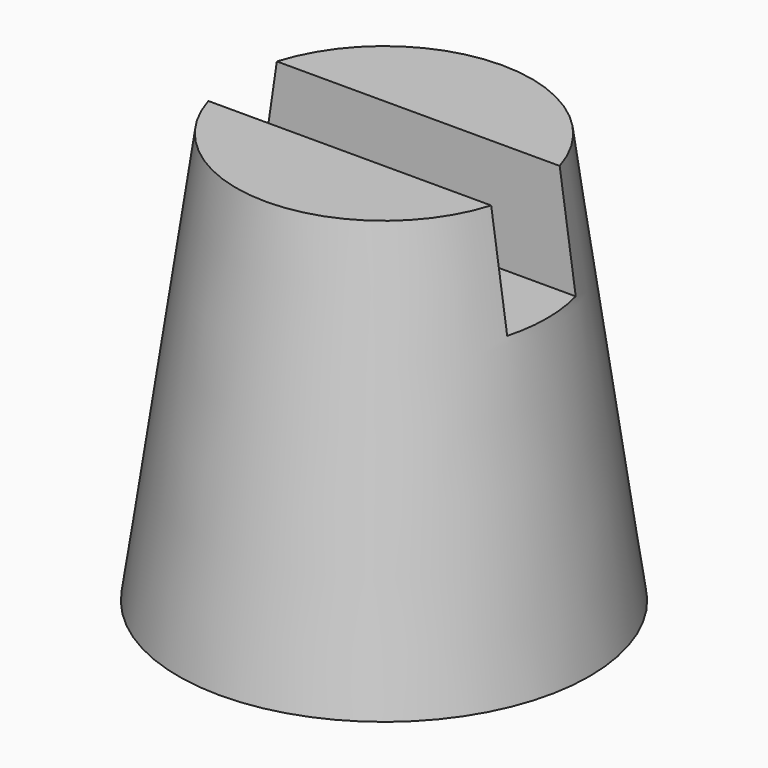
from build123d import *

# Parameters (mm, degrees)
F0_R        = 38.1
F1_DEPTH    = 76.2
F1_TAPER    = 8
F2_W        = 127
F2_H        = 15.875
F3_DEPTH    = 20.32
F4_T        = 2.5
F4_T3_DEPTH = 63.3729932057


# Not quite as in the source:
# - a shell that OpenCascade refuses in one call is made with other operations: the cavity is built on its own and cut out


with BuildPart() as f1:
    # F0 (on Top) → F1 (new body)
    with BuildSketch(Plane.XY):
        Circle(F0_R)
    extrude(amount=F1_DEPTH, taper=F1_TAPER)

    # F2 (on face) → F3 (cut)
    with BuildSketch(Plane.XY.offset(76.2)):
        Rectangle(F2_W, F2_H)
    extrude(amount=-F3_DEPTH, mode=Mode.SUBTRACT)

    # F4: shell of thickness 2.5, made by hand


with BuildPart() as f4_core1:
    # F4_t2: copy of F1
    add(f1.part)

    # the walls: a layer under each face that stays
    f4_faces = [f4_core1.faces().sort_by_distance(p)[0] for p in [
        (-32.7453941978, 0, 38.1),
        (0, 0, 55.88),
        (0, 7.9375, 66.04),
        (0, 17.6641441978, 76.2),
        (0, -7.9375, 66.04),
        (0, -17.6641441978, 76.2),
    ]]
    thicken(f4_faces, amount=-F4_T, mode=Mode.SUBTRACT)

    # F4_s4 → F4_t3 (cut)
    with BuildSketch(Plane.YZ.offset(-31.6864966028)):
        Polygon((7.9125, 55.905), (7.9375, 53.38), (10.4375, 53.38), (10.4375, 55.88), align=None)
        Polygon((-7.9125, 55.905), (-7.9375, 53.38), (-10.4375, 53.38), (-10.4375, 55.88), align=None)
    extrude(amount=F4_T3_DEPTH, mode=Mode.SUBTRACT)


with BuildPart() as f1_1:
    add(f1.part)

    # what is left inside the walls is the cavity
    f4_cavity = [f4_core1.part.solids().sort_by_distance(p)[0] for p in [
        (-32.098055, 0, 24.563187),
    ]]
    add(f4_cavity, mode=Mode.SUBTRACT)


solid = f1_1.part
